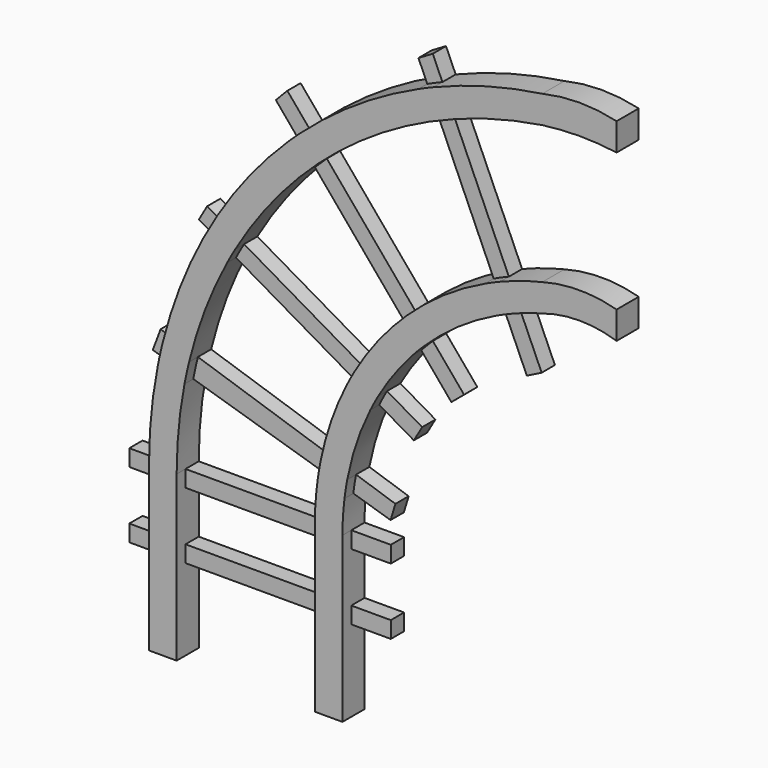
from build123d import *

# Parameters (mm, degrees)
F0_W     = 12.7
F0_H     = 7.62
F0_H_2   = 22.86
F0_H_3   = 37.4051523447
F1_DEPTH = 12.7
F2_DEPTH = 7.62
F0_W_2   = 63.5
F0_W_3   = 18.155156698
F0_W_4   = 13.1332136491


# Not quite as in the source:
# - a feature names something its author has since deleted; it is built from what else it names


with BuildPart() as f1:
    # F0 (on Front) → F1 (new body)
    with BuildSketch(Plane.XZ):
        with BuildLine():
            ThreePointArc((72.4942409164, 194.9263927655), (69.0024594084, 193.4586720894), (65.5376313263, 191.9284079148))
            Line((65.5376313263, 191.9284079149), (70.6477177027, 180.4048517764))
            ThreePointArc((70.6477177027, 180.4048517764), (74.1134811294, 181.9381956152), (77.6079402512, 183.4049658439))
            Line((77.6079402512, 183.4049658439), (72.4942409164, 194.9263927655))
        make_face()
        with BuildLine():
            ThreePointArc((65.5376313263, 191.9284079148), (37.0016277544, 176.2562354741), (11.2212317052, 156.3742921985))
            Line((11.2212317052, 156.3742921985), (19.3661217133, 146.6881956685))
            ThreePointArc((19.3661217133, 146.6881956685), (43.6934191474, 165.5443020569), (70.6477177027, 180.4048517764))
            Line((70.6477177027, 180.4048517764), (65.5376313263, 191.9284079149))
        make_face()
        with BuildLine():
            ThreePointArc((11.2212317052, 156.3742921985), (8.4251379514, 153.8042458258), (5.6758300092, 151.1842106204))
            Line((5.6758300092, 151.1842106204), (13.8373423029, 141.4720117292))
            ThreePointArc((13.8373423029, 141.4720117292), (16.576714261, 144.1066207095), (19.3661217133, 146.6881956685))
            Line((19.3661217133, 146.6881956685), (11.2212317052, 156.3742921985))
        make_face()
        with BuildLine():
            ThreePointArc((5.6758300092, 151.1842106204), (-13.5158939195, 129.8366114106), (-29.627188971, 106.0780670288))
            Line((-29.627188971, 106.0780670288), (-18.6588445745, 99.7196043812))
            ThreePointArc((-18.6588445745, 99.7196043812), (-3.8107707102, 121.6854529551), (13.8373423029, 141.4720117292))
            Line((13.8373423029, 141.4720117292), (5.6758300092, 151.1842106204))
        make_face()
        with BuildLine():
            ThreePointArc((-33.3450197452, 99.4255082292), (-44.1479728191, 75.8689076317), (-51.9766959327, 51.1640837862))
            Line((-51.9766959327, 51.1640837862), (-39.8851296429, 47.1783903994))
            ThreePointArc((-39.8851296429, 47.1783903994), (-32.5535706037, 70.6649596041), (-22.367408411, 93.061673442))
            Line((-22.367408411, 93.061673442), (-33.3450197452, 99.4255082292))
        make_face()
        with BuildLine():
            ThreePointArc((-29.627188971, 106.0780670288), (-31.5161902877, 102.7686013692), (-33.3450197452, 99.4255082292))
            Line((-33.3450197452, 99.4255082292), (-22.367408411, 93.061673442))
            ThreePointArc((-22.367408411, 93.061673442), (-20.5451434477, 96.4084728186), (-18.6588445745, 99.7196043812))
            Line((-18.6588445745, 99.7196043812), (-29.627188971, 106.0780670288))
        make_face()
        with BuildLine():
            ThreePointArc((-51.9766959327, 51.1640837862), (-53.1450685653, 46.248047274), (-54.1951949992, 41.3054018214))
            Line((-54.1951949992, 41.3054018214), (-41.9864630198, 37.5859648238))
            ThreePointArc((-41.9864630198, 37.5859648238), (-40.9952369655, 42.3951987799), (-39.8851296429, 47.1783903994))
            Line((-39.8851296429, 47.1783903994), (-51.9766959327, 51.1640837862))
        make_face()
        with BuildLine():
            ThreePointArc((-54.1951949992, 41.3054018214), (-57.2596125415, 20.7536616508), (-58.2844086191, 0))
            Line((-58.2844086191, 0), (-45.5844086191, 0))
            ThreePointArc((-45.5844086191, 0), (-44.6828710128, 18.878890091), (-41.9864630198, 37.5859648238))
            Line((-41.9864630198, 37.5859648238), (-54.1951949992, 41.3054018214))
        make_face()
        with Locations((-51.9344086191, -3.81)):
            Rectangle(F0_W, F0_H)
        with Locations((-51.9344086191, -19.05)):
            Rectangle(F0_W, F0_H_2)
        with Locations((-51.9344086191, -34.29)):
            Rectangle(F0_W, F0_H)
        with Locations((-51.9344086191, -56.8025761724)):
            Rectangle(F0_W, F0_H_3)
        with BuildLine():
            ThreePointArc((122.4739893423, 208.5260311676), (97.0645374159, 203.2681933003), (72.4942409164, 194.9263927655))
            Line((72.4942409164, 194.9263927655), (77.6079402512, 183.4049658439))
            ThreePointArc((77.6079402512, 183.4049658439), (99.6748636508, 190.9378900686), (122.4739893423, 195.8260311676))
            ThreePointArc((122.4739893423, 195.8260311676), (139.546217727, 196.9914185386), (156.6184461117, 195.8260311676))
            Line((156.6184461117, 195.8260311676), (156.6184461117, 208.5260311676))
            ThreePointArc((156.6184461117, 208.5260311676), (139.546217727, 210.5112552188), (122.4739893423, 208.5260311676))
        make_face()
    extrude(amount=F1_DEPTH)


with BuildPart() as f1b:
    # F0 (on Front) → F1, piece 2 (new body)
    with BuildSketch(Plane.XZ):
        with Locations((24.2655913809, -56.8025761724)):
            Rectangle(F0_W, F0_H_3)
        with Locations((24.2655913809, -34.29)):
            Rectangle(F0_W, F0_H)
        with Locations((24.2655913809, -19.05)):
            Rectangle(F0_W, F0_H_2)
        with Locations((24.2655913809, -3.81)):
            Rectangle(F0_W, F0_H)
        with BuildLine():
            ThreePointArc((19.2397930737, 18.9331512044), (18.2470456692, 9.4897013211), (17.9155913809, 0))
            Line((17.9155913809, 0), (30.6155913809, 0))
            ThreePointArc((30.6155913809, 0), (30.8494026067, 7.6057686039), (31.5499532863, 15.1828137067))
            Line((31.5499532863, 15.1828137067), (19.2397930737, 18.9331512044))
        make_face()
        with BuildLine():
            ThreePointArc((20.6669294611, 27.21886359), (19.889322805, 23.0870374228), (19.2397930737, 18.9331512044))
            Line((19.2397930737, 18.9331512044), (31.5499532863, 15.1828137067))
            ThreePointArc((31.5499532863, 15.1828137067), (32.1147366253, 19.2096248645), (32.8114341876, 23.2157203235))
            Line((32.8114341876, 23.2157203235), (20.6669294611, 27.21886359))
        make_face()
        with BuildLine():
            ThreePointArc((32.4919457912, 61.2591386238), (25.447107613, 44.6323534192), (20.6669294611, 27.21886359))
            Line((20.6669294611, 27.21886359), (32.8114341876, 23.2157203235))
            ThreePointArc((32.8114341876, 23.2157203235), (37.0583164786, 39.4208769095), (43.4537567697, 54.9044634661))
            Line((43.4537567697, 54.9044634661), (32.4919457912, 61.2591386238))
        make_face()
        with BuildLine():
            ThreePointArc((36.1148866878, 67.9667060665), (34.2564125864, 64.6383103056), (32.4919457912, 61.2591386238))
            Line((32.4919457912, 61.2591386238), (43.4537567697, 54.9044634661))
            ThreePointArc((43.4537567697, 54.9044634661), (45.1968150381, 58.2955203417), (47.0434534726, 61.6313029116))
            Line((47.0434534726, 61.6313029116), (36.1148866878, 67.9667060665))
        make_face()
        with BuildLine():
            ThreePointArc((54.6214602506, 92.9389150609), (44.6524873709, 80.9831960585), (36.1148866878, 67.9667060665))
            Line((36.1148866878, 67.9667060665), (47.0434534726, 61.6313029116))
            ThreePointArc((47.0434534726, 61.6313029116), (54.3222888557, 72.8619114894), (62.770670361, 83.2413557666))
            Line((62.770670361, 83.2413557666), (54.6214602506, 92.9389150609))
        make_face()
        with BuildLine():
            ThreePointArc((59.9971237765, 98.368843571), (57.2711548919, 95.6916353072), (54.6214602506, 92.9389150609))
            Line((54.6214602506, 92.9389150609), (62.770670361, 83.2413557666))
            ThreePointArc((62.770670361, 83.2413557666), (65.3872102359, 86.0347733319), (68.0888364524, 88.7459867866))
            Line((68.0888364524, 88.7459867866), (59.9971237765, 98.368843571))
        make_face()
        with BuildLine():
            ThreePointArc((96.0636950561, 123.0902742387), (77.0304705935, 112.18838891), (59.9971237765, 98.368843571))
            Line((59.9971237765, 98.368843571), (68.0888364524, 88.7459867866))
            ThreePointArc((68.0888364524, 88.7459867866), (83.6519038691, 101.5941590296), (101.0953572064, 111.7435695085))
            Line((101.0953572064, 111.7435695085), (96.0636950561, 123.0902742387))
        make_face()
        with BuildLine():
            ThreePointArc((103.0289772526, 126.1300654418), (99.5251010591, 124.6588272712), (96.0636950561, 123.0902742387))
            Line((96.0636950561, 123.0902742387), (101.0953572064, 111.7435695085))
            ThreePointArc((101.0953572064, 111.7435695085), (104.5514704754, 113.3287283392), (108.0546248268, 114.8070236535))
            Line((108.0546248268, 114.8070236535), (103.0289772526, 126.1300654418))
        make_face()
        with BuildLine():
            ThreePointArc((122.4739893423, 132.3260311676), (112.6351089689, 129.5932698578), (103.0289772526, 126.1300654418))
            Line((103.0289772526, 126.1300654418), (108.0546248268, 114.8070236535))
            ThreePointArc((108.0546248268, 114.8070236535), (115.1902758969, 117.4380424584), (122.4739893423, 119.6260311676))
            ThreePointArc((122.4739893423, 119.6260311676), (139.546217727, 122.3227880164), (156.6184461117, 119.6260311676))
            Line((156.6184461117, 119.6260311676), (156.6184461117, 132.3260311676))
            ThreePointArc((156.6184461117, 132.3260311676), (139.546217727, 134.614412379), (122.4739893423, 132.3260311676))
        make_face()
    extrude(amount=F1_DEPTH)


with BuildPart() as f2:
    # F0 (on Front) → F2 (new body)
    with BuildSketch(Plane.XZ):
        with BuildLine():
            ThreePointArc((77.6079402512, 183.4049658439), (74.1134811294, 181.9381956152), (70.6477177027, 180.4048517764))
            Line((70.6477177027, 180.4048517764), (96.0636950561, 123.0902742387))
            ThreePointArc((96.0636950561, 123.0902742387), (99.5251010591, 124.6588272712), (103.0289772526, 126.1300654418))
            Line((103.0289772526, 126.1300654418), (77.6079402512, 183.4049658439))
        make_face()
    extrude(amount=F2_DEPTH)


with BuildPart() as f2b:
    # F0 (on Front) → F2, piece 2 (new body)
    with BuildSketch(Plane.XZ):
        with BuildLine():
            ThreePointArc((19.3661217133, 146.6881956685), (16.576714261, 144.1066207095), (13.8373423029, 141.4720117292))
            Line((13.8373423029, 141.4720117292), (54.6214602506, 92.9389150609))
            ThreePointArc((54.6214602506, 92.9389150609), (57.2711548919, 95.6916353072), (59.9971237765, 98.368843571))
            Line((59.9971237765, 98.368843571), (19.3661217133, 146.6881956685))
        make_face()
    extrude(amount=F2_DEPTH)


with BuildPart() as f2c:
    # F0 (on Front) → F2, piece 3 (new body)
    with BuildSketch(Plane.XZ):
        with BuildLine():
            ThreePointArc((-18.6588445745, 99.7196043812), (-20.5451434477, 96.4084728186), (-22.367408411, 93.061673442))
            Line((-22.367408411, 93.061673442), (32.4919457912, 61.2591386238))
            ThreePointArc((32.4919457912, 61.2591386238), (34.2564125864, 64.6383103056), (36.1148866878, 67.9667060665))
            Line((36.1148866878, 67.9667060665), (-18.6588445745, 99.7196043812))
        make_face()
    extrude(amount=F2_DEPTH)


with BuildPart() as f2d:
    # F0 (on Front) → F2, piece 4 (new body)
    with BuildSketch(Plane.XZ):
        with BuildLine():
            ThreePointArc((-39.8851296429, 47.1783903994), (-40.9952369655, 42.3951987799), (-41.9864630198, 37.5859648238))
            Line((-41.9864630198, 37.5859648238), (19.2397930737, 18.9331512044))
            ThreePointArc((19.2397930737, 18.9331512044), (19.889322805, 23.0870374228), (20.6669294611, 27.21886359))
            Line((20.6669294611, 27.21886359), (-39.8851296429, 47.1783903994))
        make_face()
    extrude(amount=F2_DEPTH)


with BuildPart() as f2e:
    # F0 (on Front) → F2, piece 5 (new body)
    with BuildSketch(Plane.XZ):
        with Locations((-13.8344086191, -3.81)):
            Rectangle(F0_W_2, F0_H)
    extrude(amount=F2_DEPTH)


with BuildPart() as f2f:
    # F0 (on Front) → F2, piece 6 (new body)
    with BuildSketch(Plane.XZ):
        with Locations((-13.8344086191, -34.29)):
            Rectangle(F0_W_2, F0_H)
    extrude(amount=F2_DEPTH)


with BuildPart() as f2g:
    # F0 (on Front) → F2, piece 7 (new body)
    with BuildSketch(Plane.XZ):
        with Locations((39.6931697298, -34.29)):
            Rectangle(F0_W_3, F0_H)
    extrude(amount=F2_DEPTH)


with BuildPart() as f2h:
    # F0 (on Front) → F2, piece 8 (new body)
    with BuildSketch(Plane.XZ):
        with Locations((39.6931697298, -3.81)):
            Rectangle(F0_W_3, F0_H)
    extrude(amount=F2_DEPTH)


with BuildPart() as f2i:
    # F0 (on Front) → F2, piece 9 (new body)
    with BuildSketch(Plane.XZ):
        with BuildLine():
            ThreePointArc((32.8114341876, 23.2157203235), (32.1147366253, 19.2096248645), (31.5499532863, 15.1828137067))
            Line((31.5499532863, 15.1828137067), (48.6687680951, 9.9675011532))
            Line((48.6687680951, 9.9675011532), (50.8894609828, 17.2567345215))
            Line((50.8894609828, 17.2567345215), (32.8114341876, 23.2157203235))
        make_face()
    extrude(amount=F2_DEPTH)


with BuildPart() as f2j:
    # F0 (on Front) → F2, piece 10 (new body)
    with BuildSketch(Plane.XZ):
        with BuildLine():
            ThreePointArc((47.0434534726, 61.6313029116), (45.1968150381, 58.2955203417), (43.4537567697, 54.9044634661))
            Line((43.4537567697, 54.9044634661), (59.358157964, 45.6845176592))
            Line((59.358157964, 45.6845176592), (63.1798208408, 52.2768839154))
            Line((63.1798208408, 52.2768839154), (47.0434534726, 61.6313029116))
        make_face()
    extrude(amount=F2_DEPTH)


with BuildPart() as f2k:
    # F0 (on Front) → F2, piece 11 (new body)
    with BuildSketch(Plane.XZ):
        with BuildLine():
            ThreePointArc((68.0888364524, 88.7459867866), (65.3872102359, 86.0347733319), (62.770670361, 83.2413557666))
            Line((62.770670361, 83.2413557666), (76.5995979309, 66.7849332094))
            Line((76.5995979309, 66.7849332094), (82.4333029651, 71.6872067201))
            Line((82.4333029651, 71.6872067201), (68.0888364524, 88.7459867866))
        make_face()
    extrude(amount=F2_DEPTH)


with BuildPart() as f2l:
    # F0 (on Front) → F2, piece 12 (new body)
    with BuildSketch(Plane.XZ):
        with BuildLine():
            ThreePointArc((108.0546248268, 114.8070236535), (104.5514704754, 113.3287283392), (101.0953572064, 111.7435695085))
            Line((101.0953572064, 111.7435695085), (111.2848296762, 88.7656882405))
            Line((111.2848296762, 88.7656882405), (118.1003655521, 92.1734544771))
            Line((118.1003655521, 92.1734544771), (108.0546248268, 114.8070236535))
        make_face()
    extrude(amount=F2_DEPTH)


with BuildPart() as f2m:
    # F0 (on Front) → F2, piece 13 (new body)
    with BuildSketch(Plane.XZ):
        with BuildLine():
            Line((61.475224793, 201.0893821716), (65.5376313263, 191.9284079149))
            ThreePointArc((65.5376313263, 191.9284079148), (69.0024594084, 193.4586720894), (72.4942409164, 194.9263927655))
            Line((72.4942409164, 194.9263927655), (68.0468335916, 204.9466296095))
            Line((68.0468335916, 204.9466296095), (61.475224793, 201.0893821716))
        make_face()
    extrude(amount=F2_DEPTH)


with BuildPart() as f2n:
    # F0 (on Front) → F2, piece 14 (new body)
    with BuildSketch(Plane.XZ):
        with BuildLine():
            Line((-4.063737113, 162.7742946148), (5.6758300092, 151.1842106204))
            ThreePointArc((5.6758300092, 151.1842106204), (8.4251379514, 153.8042458258), (11.2212317052, 156.3742921985))
            Line((11.2212317052, 156.3742921985), (1.2338773265, 168.251491092))
            Line((1.2338773265, 168.251491092), (-4.063737113, 162.7742946148))
        make_face()
    extrude(amount=F2_DEPTH)


with BuildPart() as f2o:
    # F0 (on Front) → F2, piece 15 (new body)
    with BuildSketch(Plane.XZ):
        with BuildLine():
            Line((-39.4252841529, 102.9503003699), (-33.3450197452, 99.4255082292))
            ThreePointArc((-33.3450197452, 99.4255082292), (-31.5161902877, 102.7686013692), (-29.627188971, 106.0780670288))
            Line((-29.627188971, 106.0780670288), (-35.6036212762, 109.5426666261))
            Line((-35.6036212762, 109.5426666261), (-39.4252841529, 102.9503003699))
        make_face()
    extrude(amount=F2_DEPTH)


with BuildPart() as f2p:
    # F0 (on Front) → F2, piece 16 (new body)
    with BuildSketch(Plane.XZ):
        with BuildLine():
            Line((-60.6135897692, 43.2607903919), (-54.1951949992, 41.3054018214))
            ThreePointArc((-54.1951949992, 41.3054018214), (-53.1450685653, 46.248047274), (-51.9766959327, 51.1640837862))
            Line((-51.9766959327, 51.1640837862), (-57.0226085548, 52.8273472615))
            Line((-57.0226085548, 52.8273472615), (-60.6135897692, 43.2607903919))
        make_face()
    extrude(amount=F2_DEPTH)


with BuildPart() as f2q:
    # F0 (on Front) → F2, piece 17 (new body)
    with BuildSketch(Plane.XZ):
        with Locations((-64.8510154437, -3.81)):
            Rectangle(F0_W_4, F0_H)
    extrude(amount=F2_DEPTH)


with BuildPart() as f2r:
    # F0 (on Front) → F2, piece 18 (new body)
    with BuildSketch(Plane.XZ):
        with Locations((-64.8510154437, -34.29)):
            Rectangle(F0_W_4, F0_H)
    extrude(amount=F2_DEPTH)


solid = Compound([f1.part, f1b.part, f2.part, f2b.part, f2c.part, f2d.part, f2e.part, f2f.part, f2g.part, f2h.part, f2i.part, f2j.part, f2k.part, f2l.part, f2m.part, f2n.part, f2o.part, f2p.part, f2q.part, f2r.part])
